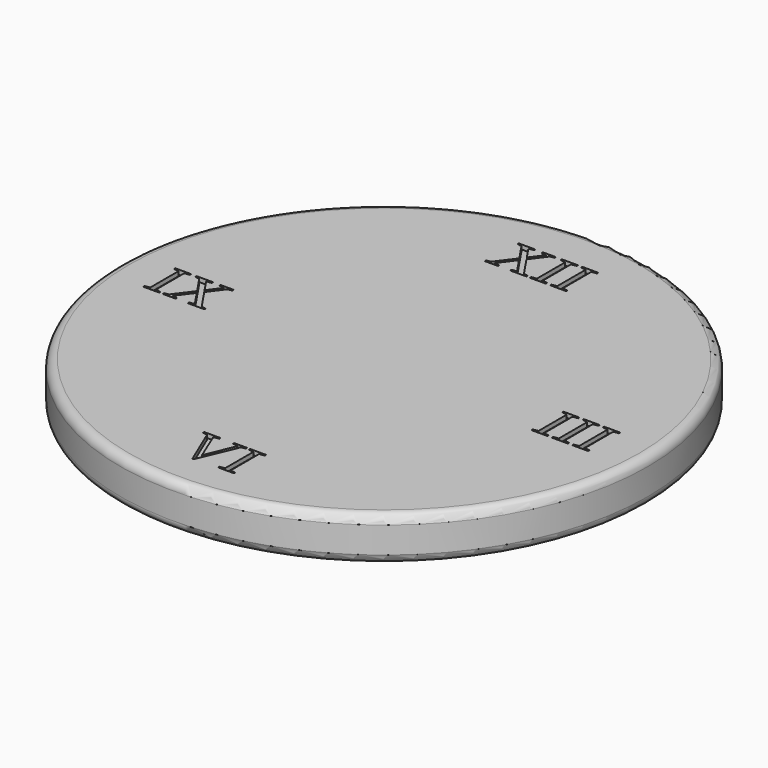
from build123d import *

# Parameters (mm, degrees)
F0_R         = 152.4
F1_DEPTH     = 25.4
F2_R         = 5.08
F3_TEXT_SIZE = 35.2777777778
F4_DEPTH     = 2.54


# Not quite as in the source:
# - Text() gives the source's letters only with a copy of the font that has no kerning and outlines rounded to 1/6400 em; it was checked with that copy


with BuildPart() as f1:
    # F0 (on Top) → F1 (new body)
    with BuildSketch(Plane.XY):
        Circle(F0_R)
    extrude(amount=F1_DEPTH)

    # F2
    f2_edges = [f1.edges().sort_by_distance(p)[0] for p in [
        (-152.4, 0, 25.4),
        (-152.4, 0, 0),
    ]]
    fillet(f2_edges, radius=F2_R)

    # F3 (on face) → F4 (cut)
    with BuildSketch(Plane.XY.offset(25.4)):
        with Locations((-24.9672960069, 103.0051799193)):
            Text('XII', F3_TEXT_SIZE, font='Tinos', text_align=(TextAlign.LEFT, TextAlign.BOTTOM))
        with Locations((93.9882160262, -12.7)):
            Text('III', F3_TEXT_SIZE, font='Tinos', text_align=(TextAlign.LEFT, TextAlign.BOTTOM))
        with Locations((-19.0940972222, -129.4089314973)):
            Text('VI', F3_TEXT_SIZE, font='Tinos', text_align=(TextAlign.LEFT, TextAlign.BOTTOM))
        with Locations((-130.1920354707, -12.7)):
            Text('IX', F3_TEXT_SIZE, font='Tinos', text_align=(TextAlign.LEFT, TextAlign.BOTTOM))
    extrude(amount=-F4_DEPTH, mode=Mode.SUBTRACT)


solid = f1.part
